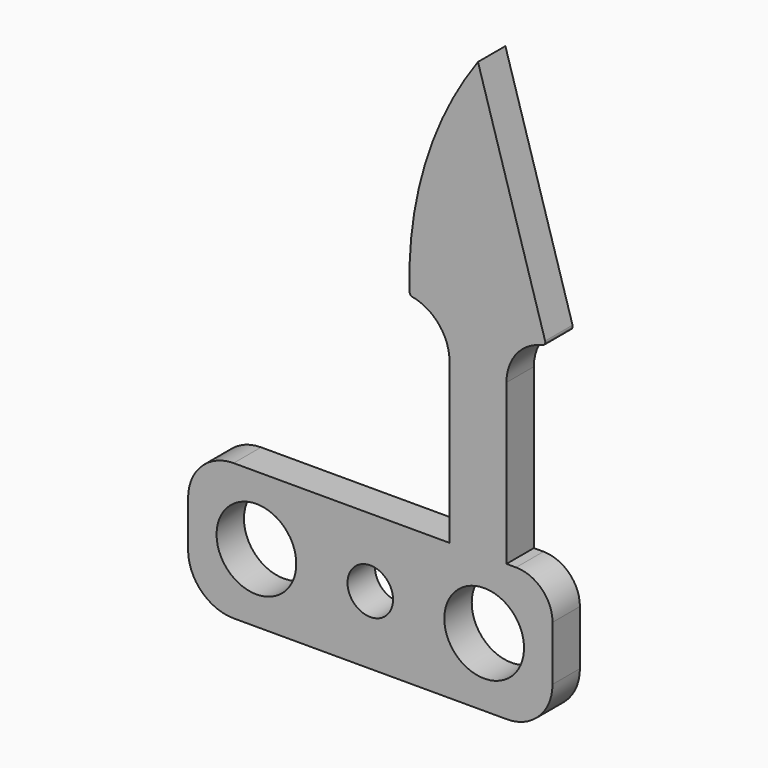
from build123d import *

# Parameters (mm, degrees)
F1_W           = 50.8
F1_H           = 19.05
F2_DEPTH       = 2.3876
F2_DEPTH_BACK  = 2.3876
F3_R           = 5.08
F4_R           = 6.35
F5_R           = 6.35
F7_D           = 11.1125
F9_D           = 11.1125
F11_D          = 6.35
F13_DEPTH      = 2.3876
F13_DEPTH_BACK = 2.3876
F15_DEPTH      = 2.3876
F15_DEPTH_BACK = 2.3876
F16_T1_DEPTH   = 4.7752
F16_T6_DEPTH   = 4.7752
F17_R          = 0.508


# Not quite as in the source:
# - a fillet or chamfer that OpenCascade refuses, or shapes differently, is made with other operations: its cross-section is extruded or revolved along the edge and cut away or added


with BuildPart() as f2:
    # F1 (on face) → F2 (new body, two sides)
    with BuildSketch(Plane.XZ) as f2_sk:
        with Locations((-6.4059151608, 1.9555166364)):
            Rectangle(F1_W, F1_H)
    extrude(amount=F2_DEPTH)
    extrude(f2_sk.sketch, amount=-F2_DEPTH_BACK)

    # F3
    f3_edges = [f2.edges().sort_by_distance(p)[0] for p in [
        (18.994085, 0, 11.480517),
    ]]
    fillet(f3_edges, radius=F3_R)

    # F4
    f4_edges = [f2.edges().sort_by_distance(p)[0] for p in [
        (18.994085, 0, -7.569483),
    ]]
    fillet(f4_edges, radius=F4_R)

    # F5
    f5_edges = [f2.edges().sort_by_distance(p)[0] for p in [
        (-31.805915, 0, 11.480517),
        (-31.805915, 0, -7.569483),
    ]]
    fillet(f5_edges, radius=F5_R)

    # F7 (through all)
    with Locations(Plane.XZ.offset(2.3876)):
        with Locations((9.4690848392, 1.9555166364)):
            Hole(F7_D / 2)

    # F9 (through all)
    with Locations(Plane.XZ.offset(2.3876)):
        with Locations((-22.2809151608, 1.9555166364)):
            Hole(F9_D / 2)

    # F11 (through all)
    with Locations(Plane.XZ.offset(2.3876)):
        with Locations((-6.4059151608, 1.9555166364)):
            Hole(F11_D / 2)

    # F12 (on Front) → F13 (join, two sides)
    with BuildSketch(Plane.XZ) as f13_sk:
        Polygon((8.6054187268, 40.0424157364), (4.6366687268, 40.0424157364), (4.6366687268, 11.4674157364), (12.5741687268, 11.4674157364), (12.5741687268, 40.0424157364), align=None)
    extrude(amount=F13_DEPTH)
    extrude(f13_sk.sketch, amount=-F13_DEPTH_BACK)

    # F14 (on Front) → F15 (join, two sides)
    with BuildSketch(Plane.XZ) as f15_sk:
        with BuildLine():
            Line((18.1304187268, 40.0424157364), (8.6054187268, 71.7924157364))
            ThreePointArc((8.6054187268, 71.7924157364), (1.180386736, 56.7161753336), (-0.9195812732, 40.0424157364))
            Line((-0.9195812732, 40.0424157364), (8.6054187268, 40.0424157364))
            Line((8.6054187268, 40.0424157364), (18.1304187268, 40.0424157364))
        make_face()
    extrude(amount=F15_DEPTH)
    extrude(f15_sk.sketch, amount=-F15_DEPTH_BACK)

    # F16: fillet of radius 6.35 on 2 edges, made by hand

    # F16_s2 → F16_t1 (join)
    with BuildSketch(Plane.XZ.offset(-2.3876)):
        with BuildLine():
            ThreePointArc((-0.9195812732, 40.0424157364), (3.0491687268, 37.9423506332), (4.6366687268, 33.7422204269))
            Line((4.6366687268, 33.7422204269), (4.7636687268, 33.7422204269))
            Line((4.7636687268, 33.7422204269), (4.7636687268, 40.0424157364))
            Line((4.7636687268, 40.0424157364), (4.6366687268, 40.1694157364))
            ThreePointArc((4.6366687268, 40.1694157364), (1.8585437268, 40.1694157364), (-0.9037062732, 40.1684196426))
            Line((-0.9037062732, 40.1684196426), (-0.9195812732, 40.0424157364))
        make_face()
    extrude(amount=F16_T1_DEPTH)


with BuildPart() as f16_tool4:
    # F16_s5 → F16_t6 (new body)
    with BuildSketch(Plane.XZ.offset(2.3876)):
        with BuildLine():
            ThreePointArc((18.1304187268, 40.0424157364), (14.1616687268, 37.9423506332), (12.5741687268, 33.7422204269))
            Line((12.5741687268, 33.7422204269), (12.4471687268, 33.7422204269))
            Line((12.4471687268, 33.7422204269), (12.4471687268, 40.0424157364))
            Line((12.4471687268, 40.0424157364), (12.5741687268, 40.1694157364))
            ThreePointArc((12.5741687268, 40.1694157364), (15.3522937268, 40.1694157364), (18.1145437268, 40.1684196426))
            Line((18.1145437268, 40.1684196426), (18.1304187268, 40.0424157364))
        make_face()
    extrude(amount=-F16_T6_DEPTH)

    split(bisect_by=Plane(origin=(27.6542600438, 0, 8.2962780131), x_dir=(0, 1, 0), z_dir=(-0.9578262852, 0, -0.2873478856)), keep=Keep.TOP)


with BuildPart() as f2_1:
    add(f2.part)

    # F16_t3: union F16_tool4
    add(f16_tool4.part)

    # F17
    f17_edges = [f2_1.edges().sort_by_distance(p)[0] for p in [
        (18.130419, 0, 40.042416),
        (-0.919581, 0, 40.042416),
    ]]
    fillet(f17_edges, radius=F17_R)


solid = f2_1.part
